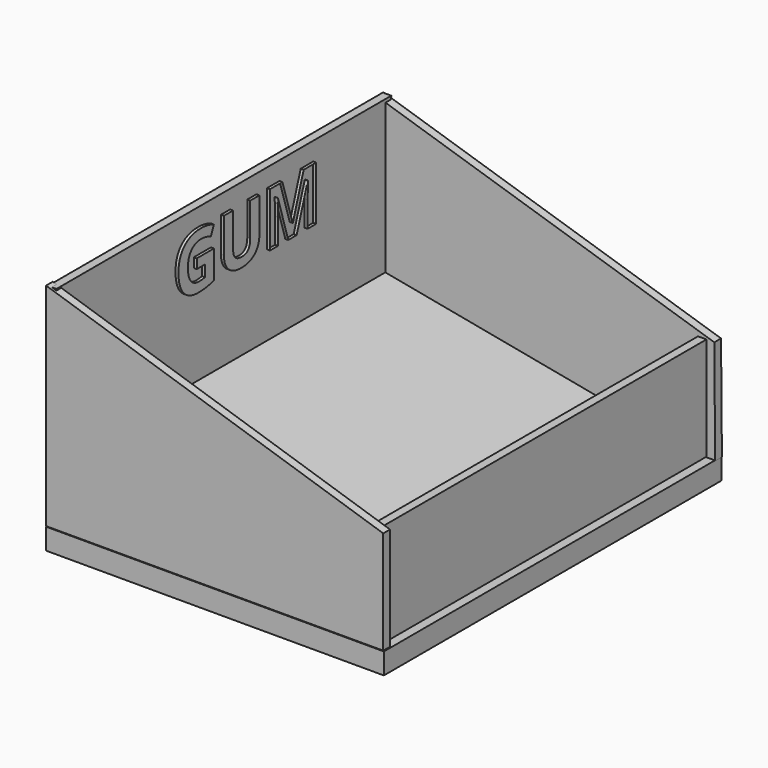
from build123d import *

# Parameters (mm, degrees)
F1_DEPTH      = 12.7
F3_DEPTH      = 5.08
F6_DEPTH      = 5.08
F9_DEPTH      = 5.08
F11_W         = 254.2360723019
F11_H         = 62.0994120836
F12_DEPTH     = 5.08
F15_DEPTH     = 241.3
F16_TEXT_SIZE = 45.504514128
F17_DEPTH     = 6.858


# Not quite as in the source:
# - Text() gives the source's letters only with a copy of the font that has no kerning and outlines rounded to 1/6400 em; it was checked with that copy


with BuildPart() as f1:
    # F0 (on Top) → F1 (new body)
    with BuildSketch(Plane.XY):
        Polygon((0, 127), (0, 0), (0, -127), (203.2, -127), (203.2, 126.7234236002), align=None)
    extrude(amount=F1_DEPTH)

    # F2 (on Right) → F3 (join)
    with BuildSketch(Plane.YZ):
        Polygon((-125.5739701088, 139.684544485), (-125.5739701088, 12.684544485), (125.5418404599, 12.684544485), (125.5418404599, 112.0610782336), (126.211471587, 139.684544485), align=None)
    extrude(amount=F3_DEPTH)

    # F5 (on offset) → F6 (join)
    with BuildSketch(Plane.XZ.offset(127)):
        Polygon((202.8254419565, 75.1166492701), (0, 140.4006481171), (0, 13.0172371864), (202.8254419565, 13.0172371864), align=None)
    extrude(amount=-F6_DEPTH)

    # F8 (on offset) → F9 (join)
    with BuildSketch(Plane.XZ.offset(-127)):
        Polygon((202.8257548809, 75.1166492701), (0, 139.3391191959), (0, 13.0172371864), (203.3565193415, 12.4864727259), align=None)
    extrude(amount=F9_DEPTH)

    # F11 (on offset) → F12 (join)
    with BuildSketch(Plane.YZ.offset(198.12)):
        with Locations((0.214189291, 44.0669432282)):
            Rectangle(F11_W, F11_H)
    extrude(amount=-F12_DEPTH)

    # F14 (on offset) → F15 (join)
    with BuildSketch(Plane.XZ.offset(120.65)):
        Polygon((5.9428415261, 48.6435070634), (5.9428415261, 12.3016834259), (167.7933782339, 12.3016834259), (198.2038021088, 12.3016834259), align=None)
    extrude(amount=-F15_DEPTH)

    # F16 (on Right) → F17 (join)
    with BuildSketch(Plane.YZ):
        with Locations((-38.6668667197, 96.221126616)):
            Text('GUM', F16_TEXT_SIZE, font='Open Sans', font_style=FontStyle.BOLD, text_align=(TextAlign.LEFT, TextAlign.BOTTOM))
    extrude(amount=F17_DEPTH)


solid = f1.part
